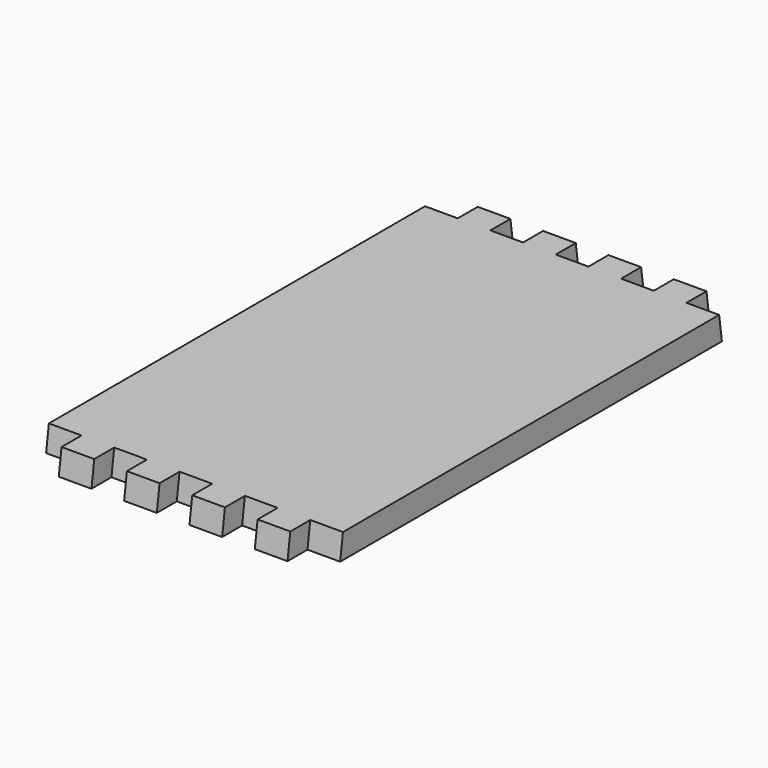
from build123d import *

# Parameters (mm, degrees)
F0_W     = 214.3125
F0_H     = 384.175
F1_DEPTH = 18.034
F3_DEPTH = 214.3125
F6_DEPTH = 18.034


# Not quite as in the source:
# - a pattern or mirror of a feature is missing from the dataset's text; its kind, count and spacing are read off the source's solid


with BuildPart() as f1:
    # F0 (on Top) → F1 (new body)
    with BuildSketch(Plane.XY):
        Rectangle(F0_W, F0_H)
    extrude(amount=F1_DEPTH)

    # F2 (on face) → F3 (cut, through all)
    with BuildSketch(Plane(origin=(-107.15625, 0, 0), x_dir=(0, -1, 0), z_dir=(-1, 0, 0))):
        Polygon((-204.7875, 0), (-192.0875, 0), (-189.552986587, 18.034), (-204.7875, 18.034), align=None)
    f3 = extrude(amount=-F3_DEPTH, mode=Mode.SUBTRACT)

    # F3_copies: F3 across plane
    add(f3.mirror(Plane(origin=(0, 0, 0), x_dir=(0, 0, -1), z_dir=(0, -1, 0))), mode=Mode.SUBTRACT)

    # F5 (on offset) → F6 (cut)
    with BuildSketch(Plane(origin=(0, 188.3669280093, 26.4732452927), x_dir=(-1, 0, 0), z_dir=(0, 0.9902680687, 0.139173101))):
        Polygon((-83.34375, -1.3334130307), (-107.15625, -1.3334130307), (-107.15625, -26.7334130307), (-107.15625, -33.0834130307), (107.15625, -33.0834130307), (107.15625, -26.7334130307), (107.15625, -1.3334130307), (83.34375, -1.3334130307), (83.34375, -26.7334130307), (59.53125, -26.7334130307), (59.53125, -1.3334130307), (35.71875, -1.3334130307), (35.71875, -26.7334130307), (11.90625, -26.7334130307), (11.90625, -1.3334130307), (-11.90625, -1.3334130307), (-11.90625, -26.7334130307), (-35.71875, -26.7334130307), (-35.71875, -1.3334130307), (-59.53125, -1.3334130307), (-59.53125, -26.7334130307), (-83.34375, -26.7334130307), align=None)
    f6 = extrude(amount=-F6_DEPTH, mode=Mode.SUBTRACT)

    # F6_copies: F6 across plane
    add(f6.mirror(Plane(origin=(0, 0, 0), x_dir=(0, 0, -1), z_dir=(0, -1, 0))), mode=Mode.SUBTRACT)


solid = f1.part
